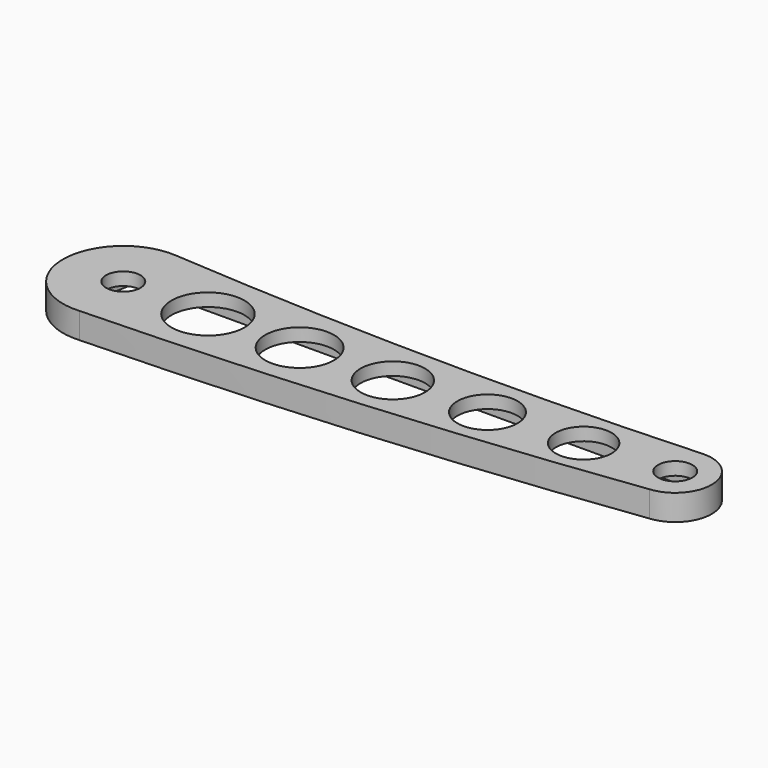
from build123d import *

# Parameters (mm, degrees)
F0_R     = 8.5
F0_R_2   = 8
F0_R_3   = 4
F0_R_4   = 7.5
F0_R_5   = 7
F0_R_6   = 6.5
F1_DEPTH = 6
F3_DEPTH = 3


# Not quite as in the source:
# - ends of sketch curves that miss each other by under 0.0002 mm in the source are joined


with BuildPart() as f1:
    # F0 (on Top) → F1 (new body)
    with BuildSketch(Plane.XY):
        with BuildLine():
            ThreePointArc((44.5540603798, 26.8468655378), (-17.2418869333, 25.5132571498), (-79.0021794007, 28))
            ThreePointArc((-79.0021794007, 28), (-94.0355137401, 14), (-79.0021794007, 0))
            ThreePointArc((-79.0021794007, 0), (-16.5001968513, 3.3088101205), (45.7422348275, 9.8910396618))
            ThreePointArc((45.7422348275, 9.8910396618), (53.4792070742, 18.9527489424), (44.5540603798, 26.8468655378))
        make_face()
        with Locations((-60.0031413922, 13.6455344589)):
            Circle(F0_R, mode=Mode.SUBTRACT)
        with Locations((-38.7143914059, 13.7077101978)):
            Circle(F0_R_2, mode=Mode.SUBTRACT)
        with Locations((-80, 14)):
            Circle(F0_R_3, mode=Mode.SUBTRACT)
        with Locations((-17.4317891816, 14.2230589801)):
            Circle(F0_R_4, mode=Mode.SUBTRACT)
        with Locations((3.8350196915, 15.191347242)):
            Circle(F0_R_5, mode=Mode.SUBTRACT)
        with Locations((25.0763967822, 16.6121361411)):
            Circle(F0_R_6, mode=Mode.SUBTRACT)
        with Locations((45, 18.3585710294)):
            Circle(F0_R_3, mode=Mode.SUBTRACT)
    extrude(amount=F1_DEPTH)

    # F2 (on Top) → F3 (cut)
    with BuildSketch(Plane.XY):
        with BuildLine():
            Line((48.3999060802, 23.8845237164), (-85.0995088492, 23.4892851738))
            ThreePointArc((-85.0995088492, 23.4892851738), (-86.3603062967, 13.0242161587), (-85.7702605867, 2.5))
            Line((-85.7702605867, 2.5), (48.4354331402, 11.884576307))
            ThreePointArc((48.4354331402, 11.884576307), (49.0927734894, 17.8865487251), (48.3999060802, 23.8845237164))
        make_face()
    extrude(amount=F3_DEPTH, mode=Mode.SUBTRACT)


solid = f1.part
